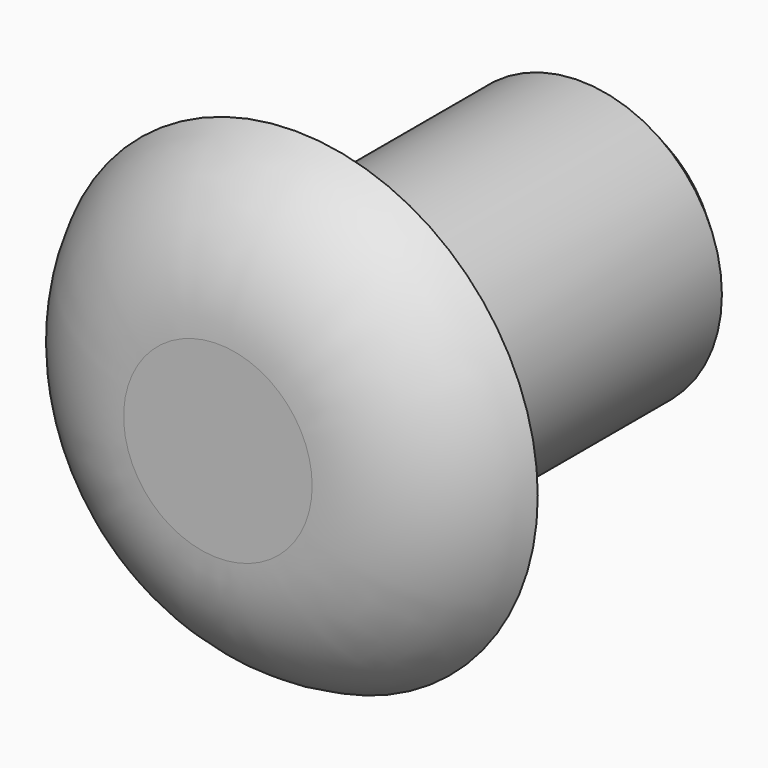
from build123d import *

# Parameters (mm, degrees)
F0_R     = 4.4
F1_DEPTH = 12
F2_R     = 7.5
F2_R_2   = 4.4
F3_DEPTH = 3
F5_SIZE  = 1


# Not quite as in the source:
# - a fillet or chamfer that OpenCascade refuses, or shapes differently, is made with other operations: its cross-section is extruded or revolved along the edge and cut away or added


with BuildPart() as f1:
    # F0 (on Front) → F1 (new body)
    with BuildSketch(Plane.XZ):
        Circle(F0_R)
    extrude(amount=F1_DEPTH)

    # F2 (on face) → F3 (join)
    with BuildSketch(Plane.XZ.offset(12)):
        Circle(F2_R)
        Circle(F2_R_2, mode=Mode.SUBTRACT)
        Circle(F2_R)
    extrude(amount=F3_DEPTH)

    # F4: fillet of radius 5 on 1 edges, made by hand

    # F4_s1 → F4_t2 (revolve, cut)
    with BuildSketch(Plane.XY):
        with BuildLine():
            ThreePointArc((7.5, -12), (5.6560370926, -14.1833001327), (2.917424305, -15))
            Line((2.917424305, -15), (7.5, -15))
            Line((7.5, -15), (7.5, -12))
        make_face()
    revolve(axis=Axis((0, -15, 0), (0, -1, 0)), mode=Mode.SUBTRACT)

    # F5
    f5_edges = [f1.edges().sort_by_distance(p)[0] for p in [
        (-4.4, 0, 0),
    ]]
    chamfer(f5_edges, length=F5_SIZE)


solid = f1.part
